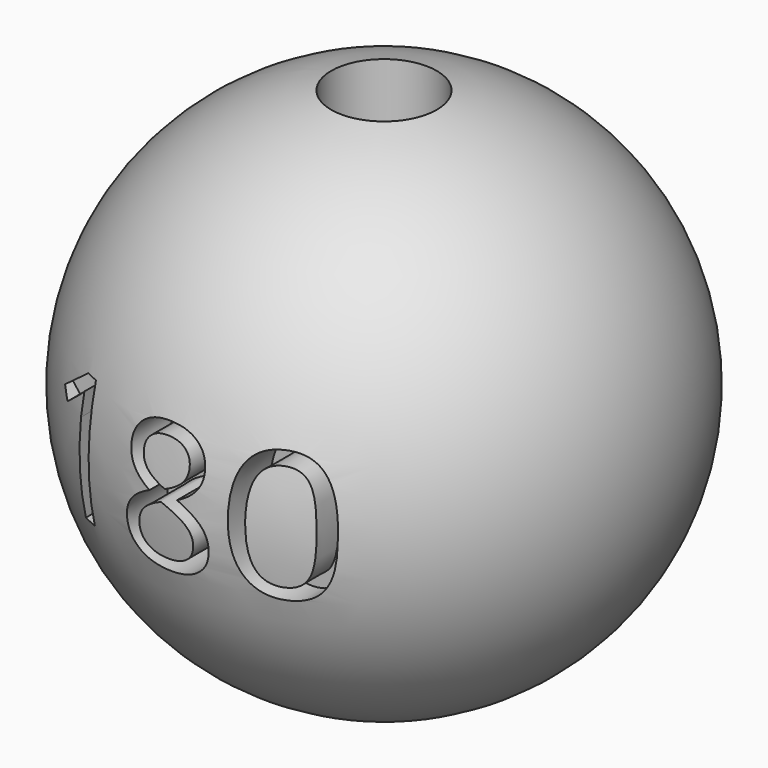
from build123d import *

# Parameters (mm, degrees)
F4_R          = 3.175
F5_DEPTH      = 9.525
F7_R          = 3.175
F8_DEPTH      = 9.525
F10_TEXT_SIZE = 10.7540322157
F11_DEPTH     = 4.064


# Not quite as in the source:
# - Text() gives the source's letters only with a copy of the font that has no kerning and outlines rounded to 1/6400 em; it was checked with that copy


with BuildPart() as f2:
    # F0 (on Front) → F2 (revolve)
    with BuildSketch(Plane.XZ):
        with BuildLine():
            Line((0, -15.875), (0, 15.875))
            ThreePointArc((0, 15.875), (-15.875, 0), (0, -15.875))
        make_face()
    revolve(axis=Axis((0, 0, 0), (0, 0, 1)))

    # F4 (on offset) → F5 (cut)
    with BuildSketch(Plane.XY.offset(16.51)):
        Circle(F4_R)
    extrude(amount=-F5_DEPTH, mode=Mode.SUBTRACT)

    # F7 (on offset) → F8 (cut)
    with BuildSketch(Plane.XY.offset(-16.51)):
        Circle(F7_R)
    extrude(amount=F8_DEPTH, mode=Mode.SUBTRACT)

    # F10 (on offset) → F11 (cut)
    with BuildSketch(Plane.XZ.offset(16.51)):
        with Locations((-9.7708079265, -3.6870966433)):
            Text('180', F10_TEXT_SIZE, font='Open Sans', text_align=(TextAlign.LEFT, TextAlign.BOTTOM))
    extrude(amount=-F11_DEPTH, mode=Mode.SUBTRACT)


solid = f2.part
